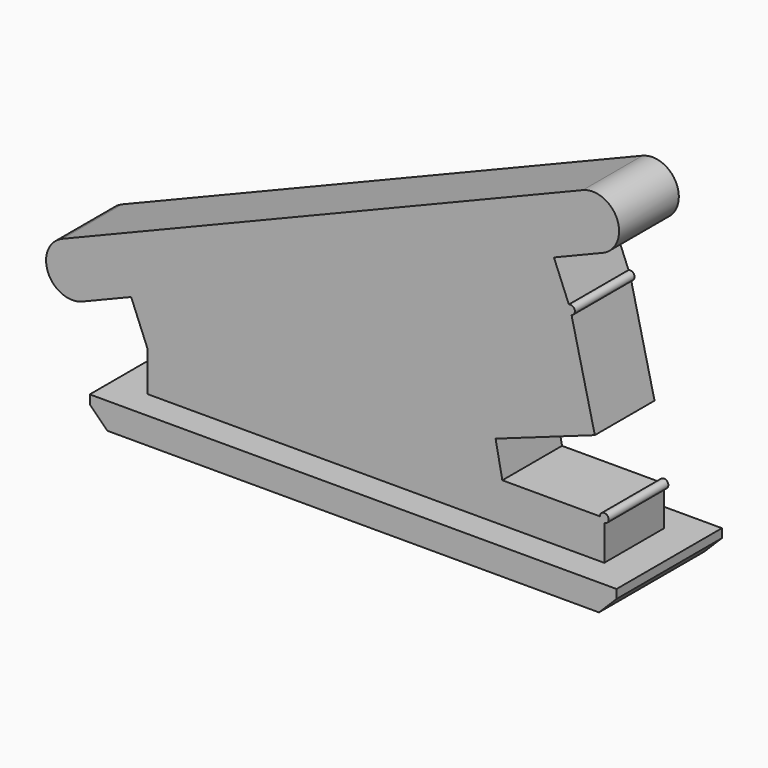
from build123d import *

# Parameters (mm, degrees)
F1_DEPTH = 3.75
F2_DEPTH = 2.125
F3_SIZE  = 1


# Not quite as in the source:
# - a feature names something its author has since deleted; it is built from what else it names


with BuildPart() as f1:
    # F0 (on Front) → F1 (new body, symmetric)
    with BuildSketch(Plane.XZ):
        Polygon((-15.2139038764, 1.5), (-15.2139038764, 0), (14.7860961236, 0), (14.7860961236, 1.5), (12.7860961236, 1.5), (-13.2139038764, 1.5), align=None)
    extrude(amount=F1_DEPTH, both=True)

    # F0 (on Front) → F2 (join, symmetric)
    with BuildSketch(Plane.XZ):
        with BuildLine():
            Line((-13.2139038764, 3.75), (-13.2139038764, 1.5))
            Line((-13.2139038764, 1.5), (12.7860961236, 1.5))
            Line((12.7860961236, 1.5), (12.7860961236, 3.5))
            ThreePointArc((12.7860961236, 3.5), (12.6093194283, 3.5732233047), (12.5360961236, 3.75))
            Line((12.5360961236, 3.75), (6.9810911579, 3.75))
            Line((6.9810911579, 3.75), (6.5964757732, 5.7126693573))
            Line((6.5964757732, 5.7126693573), (12.2487553674, 7.7255616518))
            Line((12.2487553674, 7.7255616518), (10.9207582075, 13.320105739))
            ThreePointArc((10.9207582075, 13.320105739), (10.6249391085, 13.4870718246), (10.7686600969, 13.794855662))
            Line((10.7686600969, 13.794855662), (9.9194281634, 15.8784355437))
            Line((9.9194281634, 15.8784355437), (12.6975346723, 17.0107447883))
            ThreePointArc((12.6975346723, 17.0107447883), (13.5139207983, 17.8179208397), (13.5204333045, 18.965952665))
            ThreePointArc((13.5204333045, 18.965952665), (12.713257253, 19.782338791), (11.5652254277, 19.7888512971))
            Line((11.5652254277, 19.7888512971), (-18.0679106669, 7.7108860217))
            ThreePointArc((-18.0679106669, 7.7108860217), (-18.8842967929, 6.9037099703), (-18.8908092991, 5.755678145))
            ThreePointArc((-18.8908092991, 5.755678145), (-18.0836332477, 4.939292019), (-16.9356014224, 4.9327795128))
            Line((-16.9356014224, 4.9327795128), (-14.1574949135, 6.0650887574))
            Line((-14.1574949135, 6.0650887574), (-13.2139038764, 3.75))
        make_face()
        with BuildLine():
            ThreePointArc((12.5360961236, 3.75), (12.6093194283, 3.5732233047), (12.7860961236, 3.5))
            Line((12.7860961236, 3.5), (12.7860961236, 3.75))
            Line((12.7860961236, 3.75), (12.5360961236, 3.75))
        make_face()
        with BuildLine():
            Line((12.7860961236, 3.75), (12.7860961236, 3.5))
            ThreePointArc((12.7860961236, 3.5), (12.9628728189, 3.5732233047), (13.0360961236, 3.75))
            ThreePointArc((13.0360961236, 3.75), (12.7860961236, 4), (12.5360961236, 3.75))
            Line((12.5360961236, 3.75), (12.7860961236, 3.75))
        make_face()
        with BuildLine():
            Line((10.8630192006, 13.5633467863), (10.9207582075, 13.320105739))
            ThreePointArc((10.9207582075, 13.320105739), (11.0591502177, 13.4083221943), (11.1130192006, 13.5633467863))
            ThreePointArc((11.1130192006, 13.5633467863), (11.0025007837, 13.7708194061), (10.7686600969, 13.794855662))
            Line((10.7686600969, 13.794855662), (10.8630192006, 13.5633467863))
        make_face()
        with BuildLine():
            ThreePointArc((10.7686600969, 13.794855662), (10.6249391085, 13.4870718246), (10.9207582075, 13.320105739))
            Line((10.9207582075, 13.320105739), (10.8630192006, 13.5633467863))
            Line((10.8630192006, 13.5633467863), (10.7686600969, 13.794855662))
        make_face()
    extrude(amount=F2_DEPTH, both=True)

    # F3
    f3_edges = [f1.edges().sort_by_distance(p)[0] for p in [
        (14.786096, 0, 0),
        (-15.213904, 0, 0),
    ]]
    chamfer(f3_edges, length=F3_SIZE)


solid = f1.part
